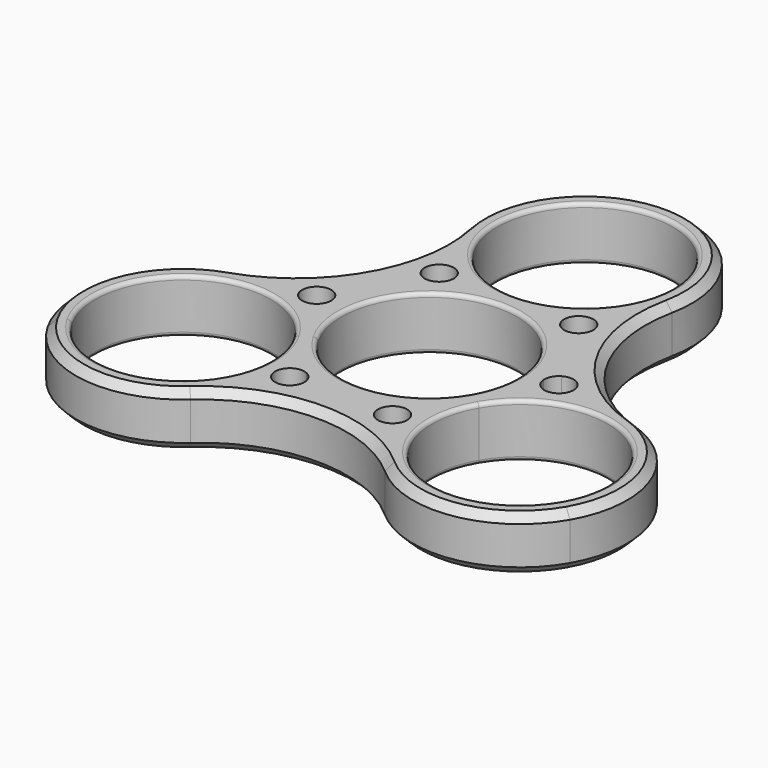
from build123d import *

# Parameters (mm, degrees)
F0_R            = 11.4681
F1_DEPTH        = 7
F2_R            = 0.508
F3_SIZE         = 1.016
F4_R            = 1.905
F5_DEPTH        = 7.001
F5_COPIES_COUNT = 3


# Not quite as in the source:
# - a pattern or mirror of a feature is missing from the dataset's text; its kind, count and spacing are read off the source's solid


with BuildPart() as f1:
    # F0 (on Top) → F1 (new body)
    with BuildSketch(Plane.XY):
        with BuildLine():
            ThreePointArc((-9.9316659331, -5.73405), (-2.9681626911, 11.0773339685), (11.4681, 0))
            ThreePointArc((11.4681, 0), (11.0773339685, -2.9681626911), (9.9316659331, -5.73405))
            Line((9.9316659331, -5.73405), (12.065379323, -6.96595))
            ThreePointArc((12.065379323, -6.96595), (24.9652079473, -1.6226660315), (33.4651452561, -12.7))
            ThreePointArc((33.4651452561, -12.7), (33.0743792246, -15.6681626911), (31.9287111893, -18.43405))
            Line((31.9287111893, -18.43405), (34.095420147, -19.685))
            ThreePointArc((34.095420147, -19.685), (35.0490813893, -7.7195127971), (26.3667546467, 0.5690067391))
            ThreePointArc((26.3667546467, 0.5690067391), (15.8276653281, 9.1381068378), (13.6761516143, 22.5497759699))
            ThreePointArc((13.6761516143, 22.5497759699), (0, 39.37), (-13.6761516143, 22.5497759699))
            ThreePointArc((-13.6761516143, 22.5497759699), (-15.8276653281, 9.1381068378), (-26.3667546467, 0.5690067391))
            ThreePointArc((-26.3667546467, 0.5690067391), (-35.0490813893, -7.7195127971), (-34.095420147, -19.685))
            Line((-34.095420147, -19.685), (-31.9287111893, -18.43405))
            ThreePointArc((-31.9287111893, -18.43405), (-27.7310952561, -2.7683340669), (-12.065379323, -6.96595))
            Line((-12.065379323, -6.96595), (-9.9316659331, -5.73405))
        make_face()
        with Locations((0, 25.4)):
            Circle(F0_R, mode=Mode.SUBTRACT)
        with BuildLine():
            ThreePointArc((9.9316659331, -5.73405), (0, -11.4681), (-9.9316659331, -5.73405))
            Line((-9.9316659331, -5.73405), (-12.065379323, -6.96595))
            ThreePointArc((-12.065379323, -6.96595), (-10.9197112877, -9.7318373089), (-10.5289452561, -12.7))
            ThreePointArc((-10.5289452561, -12.7), (-19.028882565, -23.7773339685), (-31.9287111893, -18.43405))
            Line((-31.9287111893, -18.43405), (-34.095420147, -19.685))
            ThreePointArc((-34.095420147, -19.685), (-24.2098348818, -26.4936384639), (-12.6906030324, -23.1187827089))
            ThreePointArc((-12.6906030324, -23.1187827089), (0, -18.2762136757), (12.6906030324, -23.1187827089))
            ThreePointArc((12.6906030324, -23.1187827089), (24.2098348818, -26.4936384639), (34.095420147, -19.685))
            Line((34.095420147, -19.685), (31.9287111893, -18.43405))
            ThreePointArc((31.9287111893, -18.43405), (16.2629952561, -22.6316659331), (12.065379323, -6.96595))
            Line((12.065379323, -6.96595), (9.9316659331, -5.73405))
        make_face()
    extrude(amount=F1_DEPTH)

    # F2
    f2_edges = [f1.edges().sort_by_distance(p)[0] for p in [
        (-31.928711, -18.43405, 7),
        (10.528945, -12.7, 7),
        (-11.4681, 25.4, 7),
        (-11.4681, 0, 7),
        (-31.928711, -18.43405, 0),
        (-11.4681, 25.4, 0),
        (-11.4681, 0, 0),
        (10.528945, -12.7, 0),
    ]]
    fillet(f2_edges, radius=F2_R)

    # F3
    f3_edges = [f1.edges().sort_by_distance(p)[0] for p in [
        (-15.827665, 9.138107, 7),
        (-15.827665, 9.138107, 0),
        (15.827665, 9.138107, 0),
        (0, 39.37, 0),
        (-34.09542, -19.685, 0),
        (0, -18.276214, 0),
        (34.09542, -19.685, 0),
        (15.827665, 9.138107, 7),
        (0, 39.37, 7),
        (-34.09542, -19.685, 7),
        (0, -18.276214, 7),
        (34.09542, -19.685, 7),
    ]]
    chamfer(f3_edges, length=F3_SIZE)

    # F4 (on face) → F5 (cut, through all)
    with BuildSketch(Plane.XY.offset(7)):
        with Locations((-9.1055259271, 13.0040387031)):
            Circle(F4_R)
        with Locations((-15.8145908322, 1.3835974161)):
            Circle(F4_R)
        with BuildLine():
            ThreePointArc((-7.5141526937, -16.1141524535), (-5.6855091512, -15.9942968235), (-4.8040649051, -14.3876361192))
            ThreePointArc((-4.8040649051, -14.3876361192), (-5.1024042009, -13.3640803653), (-5.9039771165, -12.6611197849))
            Line((-5.9039771165, -12.6611197849), (-7.5141526937, -16.1141524535))
        make_face()
        with BuildLine():
            Line((-7.5141526937, -16.1141524535), (-5.9039771165, -12.6611197849))
            ThreePointArc((-5.9039771165, -12.6611197849), (-8.4355812394, -13.5825483306), (-7.5141526937, -16.1141524535))
        make_face()
    f5 = extrude(amount=-F5_DEPTH, mode=Mode.SUBTRACT)

    # F5_copies: F5 ×3 about axis
    f5_copies_axis = Axis((0, 0, 0), (0, 0, 1))
    for i in range(1, F5_COPIES_COUNT):
        add(f5.rotate(f5_copies_axis, i * 360 / F5_COPIES_COUNT), mode=Mode.SUBTRACT)


solid = f1.part
